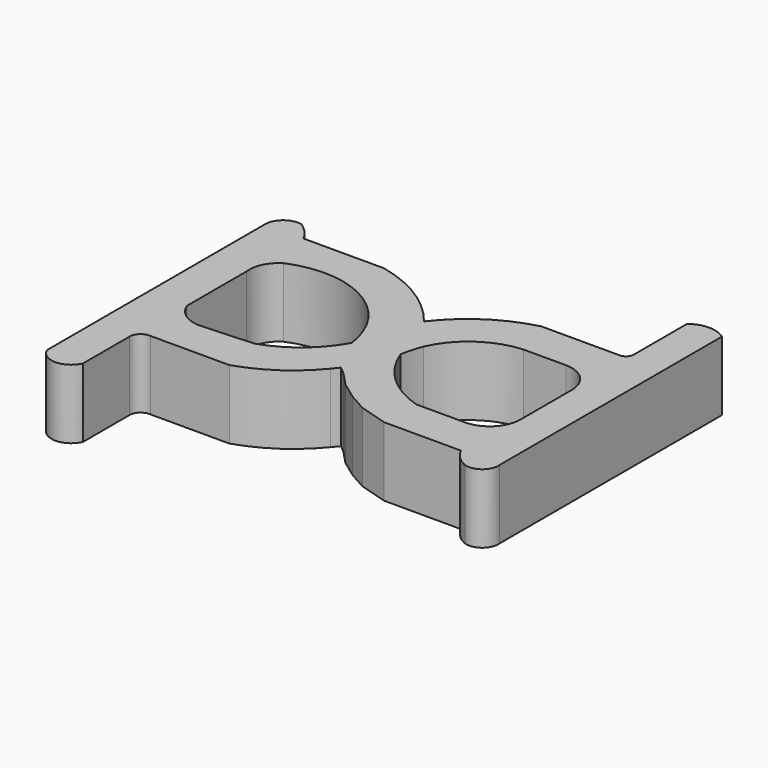
from build123d import *

# Parameters (mm, degrees)
F2_DEPTH = 25.4


# Not quite as in the source:
# - the program builds the solid bodies; features that only make, move or delete a surface that nothing else refers to are left out


with BuildPart() as f2:
    # F0 (on Top) → F2 (new body)
    with BuildSketch(Plane.XY):
        with BuildLine():
            ThreePointArc((-105.2959337831, -13.8524966314), (-110.9424227524, -15.1925239823), (-113.4453713894, -20.4283390194))
            Line((-113.4453713894, -20.4283390194), (-113.4453713894, -120.5272600055))
            ThreePointArc((-113.4453713894, -120.5272600055), (-106.8133786321, -124.9365702093), (-100.1813858747, -120.5272600055))
            Line((-100.1813858747, -120.5272600055), (-100.1813858747, -99.1557762027))
            ThreePointArc((-100.1813858747, -99.1557762027), (-98.8733273351, -96.1822516833), (-95.7974940538, -95.1372087002))
            Line((-95.7974940538, -95.1372087002), (-66.7541921139, -95.1372087002))
            ThreePointArc((-66.7541921139, -95.1372087002), (-53.508361005, -88.6629146032), (-42.6427721977, -78.6975994706))
            Line((-42.6427721977, -78.6975994706), (-40.7650305092, -76.3982318447))
            Line((-40.7650305092, -76.3982318447), (-37.9493655476, -78.6975994706))
            Line((-37.9493655476, -78.6975994706), (-33.326998353, -83.6294814944))
            Line((-33.326998353, -83.6294814944), (-27.1164793521, -88.1960391998))
            Line((-27.1164793521, -88.1960391998), (-20.3579775989, -92.0319482684))
            Line((-20.3579775989, -92.0319482684), (-9.9462270737, -95.1372087002))
            Line((-9.9462270737, -95.1372087002), (-1.5437625116, -95.1372087002))
            Line((-1.5437625116, -95.1372087002), (11.6079188883, -95.1372087002))
            Line((11.6079188883, -95.1372087002), (18.3664243668, -95.1372087002))
            ThreePointArc((18.3664243668, -95.1372087002), (21.0049540589, -98.8169422623), (24.7596036643, -101.3477295637))
            ThreePointArc((24.7596036643, -101.3477295637), (30.3769038734, -100.3890234282), (32.5886048377, -95.1372087002))
            Line((32.5886048377, -95.1372087002), (32.5886048377, -83.264157176))
            Line((32.5886048377, -83.264157176), (32.5886048377, -36.867942661))
            Line((32.5886048377, -36.867942661), (32.5886048377, 6.9710011594))
            ThreePointArc((32.5886048377, 6.9710011594), (26.2081623077, 9.0786866715), (19.8277197778, 6.9710011594))
            Line((19.8277197778, 6.9710011594), (19.8277197778, -17.5057426095))
            ThreePointArc((19.8277197778, -17.5057426095), (18.7722789641, -19.7743587388), (16.3571424782, -20.4283390194))
            Line((16.3571424782, -20.4283390194), (-11.9555136189, -20.4283390194))
            ThreePointArc((-11.9555136189, -20.4283390194), (-27.5905728803, -27.3736232216), (-40.0855019689, -39.0598885715))
            ThreePointArc((-40.0855019689, -39.0598885715), (-53.2554420129, -27.1621160119), (-69.6767866611, -20.4283390194))
            Line((-69.6767866611, -20.4283390194), (-99.268078804, -20.4283390194))
            ThreePointArc((-99.268078804, -20.4283390194), (-101.8637236034, -16.7569920607), (-105.2959337831, -13.8524966314))
        make_face()
        with BuildLine():
            ThreePointArc((-94.1535308957, -35.954631865), (-64.4908309504, -37.7586891963), (-47.9399785399, -62.4406598508))
            ThreePointArc((-47.9399785399, -62.4406598508), (-57.037773934, -73.3713012414), (-69.5008059195, -80.2212381733))
            Line((-69.5008059195, -80.2212381733), (-88.1256759167, -81.2548696995))
            ThreePointArc((-88.1256759167, -81.2548696995), (-94.899092444, -79.4350063569), (-99.268078804, -73.9483833313))
            Line((-99.268078804, -73.9483833313), (-99.268078804, -46.5490445495))
            ThreePointArc((-99.268078804, -46.5490445495), (-98.2570203257, -40.5053887944), (-94.1535308957, -35.954631865))
        make_face(mode=Mode.SUBTRACT)
        with BuildLine():
            ThreePointArc((-30.4044019431, -51.2982606888), (-20.909712223, -39.8003863828), (-6.8409675732, -34.8586589098))
            Line((-6.8409675732, -34.8586589098), (8.6853252724, -34.8586589098))
            ThreePointArc((8.6853252724, -34.8586589098), (16.4998756565, -38.1334471627), (19.6450613439, -46.0010543466))
            Line((19.6450613439, -46.0010543466), (19.6450613439, -69.3818256259))
            ThreePointArc((19.6450613439, -69.3818256259), (16.328027351, -77.3898536128), (8.3199990913, -80.7068869472))
            Line((8.3199990913, -80.7068869472), (-9.5809019141, -80.7068854751))
            ThreePointArc((-9.5809019141, -80.7068854751), (-23.6431681808, -72.6575432123), (-32.5963497162, -59.1527372599))
            ThreePointArc((-32.5963497162, -59.1527372599), (-31.6935007339, -55.171603632), (-30.4044019431, -51.2982606888))
        make_face(mode=Mode.SUBTRACT)
    extrude(amount=F2_DEPTH)


solid = f2.part
